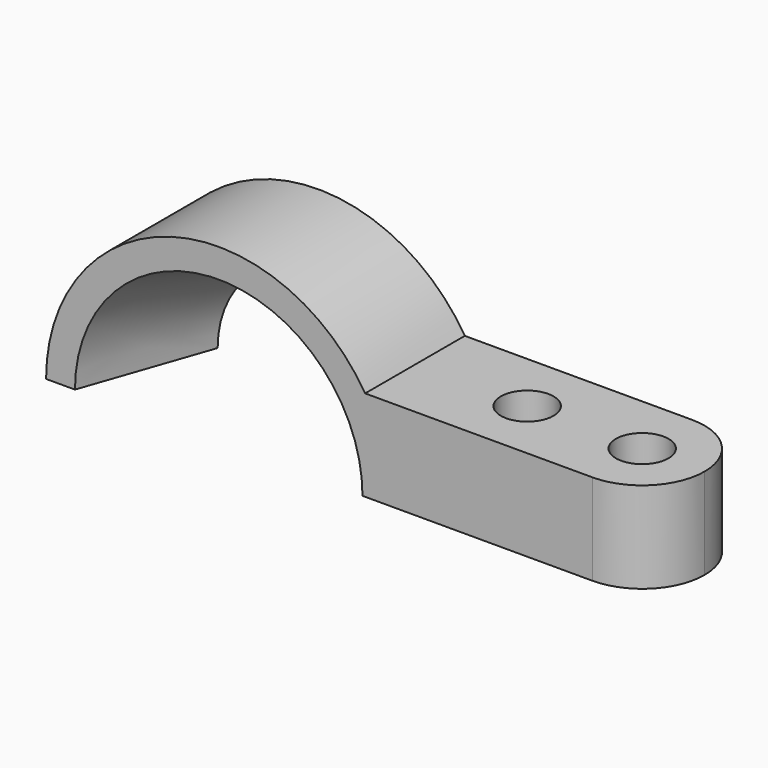
from build123d import *

# Parameters (mm, degrees)
F1_DEPTH = 52
F3_R     = 25.99999
F2_R     = 11
F4_DEPTH = 38
F5_DEPTH = 38


# Not quite as in the source:
# - a fillet or chamfer is up to 0.001 mm smaller than in the source, because OpenCascade refuses the exact size


with BuildPart() as f1:
    # F0 (on Front) → F1 (new body)
    with BuildSketch(Plane.XZ):
        with BuildLine():
            Line((46.2857175011, 0), (156.2857175011, 0))
            Line((156.2857175011, 0), (156.2857175011, 38))
            Line((156.2857175011, 38), (35.4412569068, 38))
            ThreePointArc((35.4412569068, 38), (-45.4728396677, 69.2358246763), (-97.7142824989, 0))
            Line((-97.7142824989, 0), (-67.7142824989, 0))
            ThreePointArc((-67.7142824989, 0), (-25.7142824989, 42), (16.2857175011, 0))
            Line((16.2857175011, 0), (46.2857175011, 0))
        make_face()
    extrude(amount=F1_DEPTH)

    # F3 (radius 26 in the source; OpenCascade refuses exactly that, so slightly less here)
    f3_edges = [f1.edges().sort_by_distance(p)[0] for p in [
        (156.285718, 0, 19),
        (156.285718, -52, 19),
    ]]
    fillet(f3_edges, radius=F3_R)

    # F2 (on face) → F4 (cut)
    with BuildSketch(Plane.XY.offset(38)):
        with Locations((130.2857175011, -26)):
            Circle(F2_R)
    extrude(amount=-F4_DEPTH, mode=Mode.SUBTRACT)

    # F2 (on face) → F5 (cut)
    with BuildSketch(Plane.XY.offset(38)):
        with Locations((82.2857175011, -26)):
            Circle(F2_R)
    extrude(amount=-F5_DEPTH, mode=Mode.SUBTRACT)

    # F6 (on face) → F7 (revolve, cut)
    with BuildSketch(Plane(origin=(0, 0, 0), x_dir=(1, 0, 0), z_dir=(0, 0, -1))):
        Polygon((-25.6639542129, 52), (-85.6639542129, 52), (-67.6639542129, 0), (-25.6639542129, 0), align=None)
    revolve(axis=Axis((-25.6639542129, -26, 0), (0, -1, 0)), mode=Mode.SUBTRACT)


solid = f1.part
